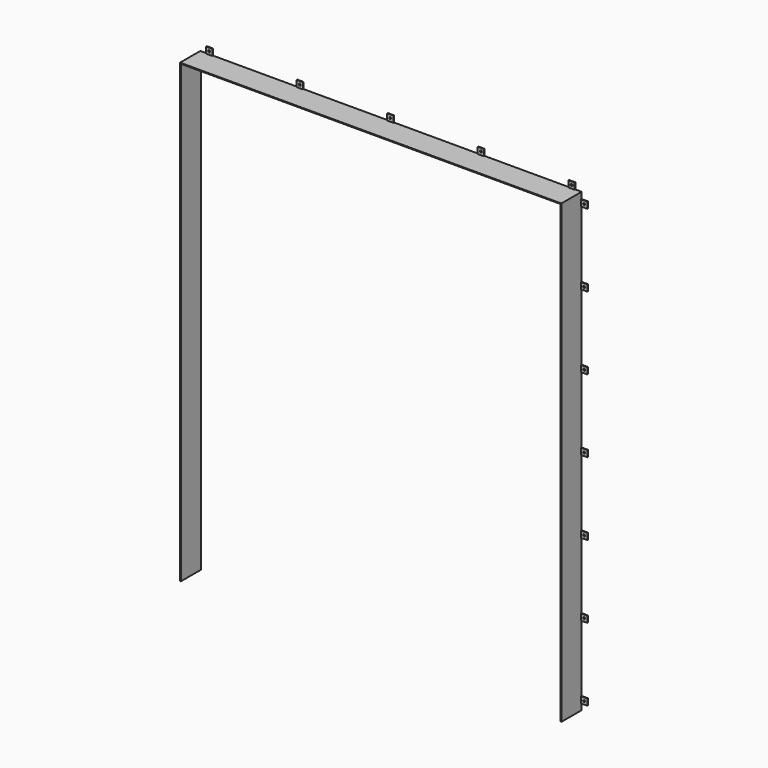
from build123d import *

# Parameters (mm, degrees)
F1_DEPTH = 101.6
F0_W     = 25.4
F0_H     = 25.4
F0_R     = 3.81
F2_DEPTH = 3.175


# Not quite as in the source:
# - a feature names something its author has since deleted; it is built from what else it names


with BuildPart() as f1:
    # F0 (on Front) → F1 (new body)
    with BuildSketch(Plane.XZ):
        Polygon((0, 25.4), (0, 0), (3.175, 0), (3.175, 1828.8), (1527.175, 1828.8), (1527.175, 0), (1530.35, 0), (1530.35, 25.4), (1530.35, 50.8), (1530.35, 318.0291666667), (1530.35, 343.4291666667), (1530.35, 610.6583333333), (1530.35, 636.0583333333), (1530.35, 903.2875), (1530.35, 928.6875), (1530.35, 1195.9166666667), (1530.35, 1221.3166666667), (1530.35, 1488.5458333333), (1530.35, 1513.9458333333), (1530.35, 1781.175), (1530.35, 1806.575), (1530.35, 1831.975), (1504.95, 1831.975), (1479.55, 1831.975), (1141.4125, 1831.975), (1116.0125, 1831.975), (777.875, 1831.975), (752.475, 1831.975), (414.3375, 1831.975), (388.9375, 1831.975), (50.8, 1831.975), (25.4, 1831.975), (0, 1831.975), (0, 1806.575), (0, 1781.175), (0, 1513.9458333333), (0, 1488.5458333333), (0, 1221.3166666667), (0, 1195.9166666667), (0, 928.6875), (0, 903.2875), (0, 636.0583333333), (0, 610.6583333333), (0, 343.4291666667), (0, 318.0291666667), (0, 50.8), align=None)
    extrude(amount=F1_DEPTH)

    # F0 (on Front) → F2 (join)
    with BuildSketch(Plane.XZ):
        with Locations((-12.7, 38.1)):
            Rectangle(F0_W, F0_H)
        with Locations((-12.7, 38.1)):
            Circle(F0_R, mode=Mode.SUBTRACT)
        with Locations((-12.7, 330.7291666667)):
            Rectangle(F0_W, F0_H)
        with Locations((-12.7, 330.7291666667)):
            Circle(F0_R, mode=Mode.SUBTRACT)
        with Locations((-12.7, 623.3583333333)):
            Rectangle(F0_W, F0_H)
        with Locations((-12.7, 623.3583333333)):
            Circle(F0_R, mode=Mode.SUBTRACT)
        with Locations((1543.05, 38.1)):
            Rectangle(F0_W, F0_H)
        with Locations((1543.05, 38.1)):
            Circle(F0_R, mode=Mode.SUBTRACT)
        with Locations((-12.7, 915.9875)):
            Rectangle(F0_W, F0_H)
        with Locations((-12.7, 915.9875)):
            Circle(F0_R, mode=Mode.SUBTRACT)
        with Locations((1543.05, 330.7291666667)):
            Rectangle(F0_W, F0_H)
        with Locations((1543.05, 330.7291666667)):
            Circle(F0_R, mode=Mode.SUBTRACT)
        with Locations((-12.7, 1208.6166666667)):
            Rectangle(F0_W, F0_H)
        with Locations((-12.7, 1208.6166666667)):
            Circle(F0_R, mode=Mode.SUBTRACT)
        with Locations((1543.05, 623.3583333333)):
            Rectangle(F0_W, F0_H)
        with Locations((1543.05, 623.3583333333)):
            Circle(F0_R, mode=Mode.SUBTRACT)
        with Locations((-12.7, 1501.2458333333)):
            Rectangle(F0_W, F0_H)
        with Locations((-12.7, 1501.2458333333)):
            Circle(F0_R, mode=Mode.SUBTRACT)
        with Locations((1543.05, 915.9875)):
            Rectangle(F0_W, F0_H)
        with Locations((1543.05, 915.9875)):
            Circle(F0_R, mode=Mode.SUBTRACT)
        with Locations((-12.7, 1793.875)):
            Rectangle(F0_W, F0_H)
        with Locations((-12.7, 1793.875)):
            Circle(F0_R, mode=Mode.SUBTRACT)
        with Locations((1543.05, 1208.6166666667)):
            Rectangle(F0_W, F0_H)
        with Locations((1543.05, 1208.6166666667)):
            Circle(F0_R, mode=Mode.SUBTRACT)
        with Locations((38.1, 1844.675)):
            Rectangle(F0_W, F0_H)
        with Locations((38.1, 1844.675)):
            Circle(F0_R, mode=Mode.SUBTRACT)
        with Locations((1543.05, 1501.2458333333)):
            Rectangle(F0_W, F0_H)
        with Locations((1543.05, 1501.2458333333)):
            Circle(F0_R, mode=Mode.SUBTRACT)
        with Locations((401.6375, 1844.675)):
            Rectangle(F0_W, F0_H)
        with Locations((401.6375, 1844.675)):
            Circle(F0_R, mode=Mode.SUBTRACT)
        with Locations((1543.05, 1793.875)):
            Rectangle(F0_W, F0_H)
        with Locations((1543.05, 1793.875)):
            Circle(F0_R, mode=Mode.SUBTRACT)
        with Locations((765.175, 1844.675)):
            Rectangle(F0_W, F0_H)
        with Locations((765.175, 1844.675)):
            Circle(F0_R, mode=Mode.SUBTRACT)
        with Locations((1492.25, 1844.675)):
            Rectangle(F0_W, F0_H)
        with Locations((1492.25, 1844.675)):
            Circle(F0_R, mode=Mode.SUBTRACT)
        with Locations((1128.7125, 1844.675)):
            Rectangle(F0_W, F0_H)
        with Locations((1128.7125, 1844.675)):
            Circle(F0_R, mode=Mode.SUBTRACT)
    extrude(amount=F2_DEPTH)


solid = f1.part
